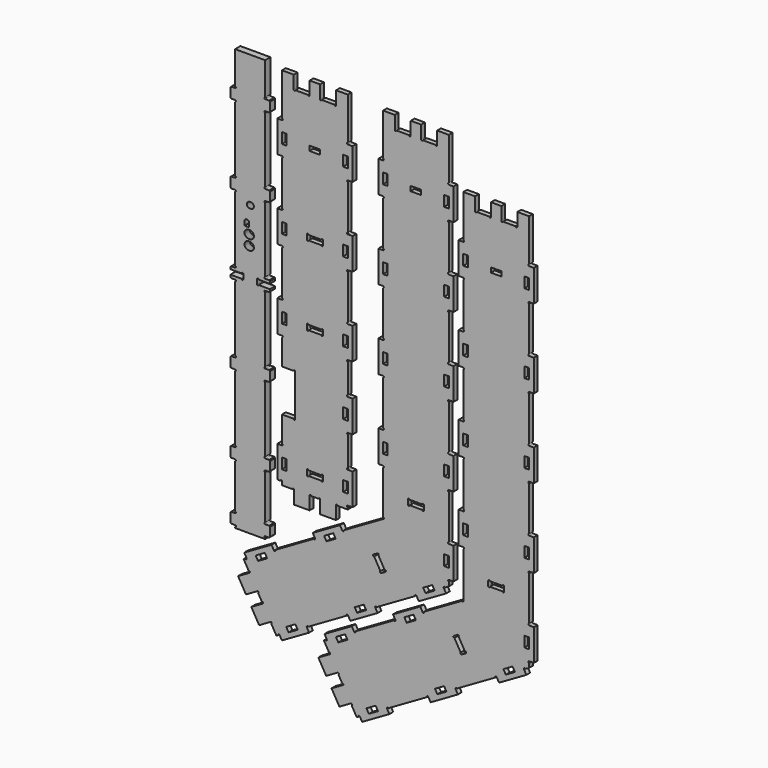
from build123d import *

# Parameters (mm, degrees)
F1_DEPTH = 25
F0_W     = 18
F0_H     = 40
F0_W_2   = 40
F0_H_2   = 18
F2_DEPTH = 18
F0_W_3   = 18.000018
F0_H_3   = 40.00004
F0_W_4   = 40.00004
F0_H_4   = 18.000018
F3_DEPTH = 18
F4_DEPTH = 18


# Not quite as in the source:
# - ends of sketch curves that miss each other by under 0.0002 mm in the source are joined


with BuildPart() as f1:
    # F0 (on Front) → F1 (new body)
    with BuildSketch(Plane.XZ):
        with BuildLine():
            Line((-423.791966, 1158.999877), (-537.792391, 1158.998909))
            Line((-537.792391, 1158.998909), (-537.791338, 1035.018779))
            ThreePointArc((-537.791338, 1035.0187789999), (-534.7813120001, 1032.0088045), (-537.791287, 1028.9987790001))
            Line((-537.791287, 1028.998779), (-552.791302, 1028.998346))
            Line((-552.791302, 1028.998346), (-555.79128, 1025.998623))
            Line((-555.79128, 1025.998623), (-555.790991, 991.998589))
            Line((-555.790991, 991.998589), (-552.790963, 988.998306))
            Line((-552.790963, 988.998306), (-537.790948, 988.998433))
            ThreePointArc((-537.790948, 988.9984329995), (-534.7808930005, 985.9884885), (-537.790837, 982.9784330005))
            Line((-537.790837, 982.978433), (-537.786301, 735.018479))
            ThreePointArc((-537.786301, 735.0184789995), (-534.7762460005, 732.008534), (-537.786191, 728.9984790005))
            Line((-537.786191, 728.998479), (-552.786206, 728.998046))
            Line((-552.786206, 728.998046), (-555.786184, 725.998323))
            Line((-555.786184, 725.998323), (-555.785895, 691.998289))
            Line((-555.785895, 691.998289), (-552.785866, 688.998006))
            Line((-552.785866, 688.998006), (-537.785851, 688.998133))
            ThreePointArc((-537.785851, 688.9981329997), (-534.7758110003, 685.988173), (-537.785771, 682.9781330003))
            Line((-537.785771, 682.978133), (-537.78245, 435.016937))
            ThreePointArc((-537.78245, 435.0169369997), (-534.7724100003, 432.0069775), (-537.782369, 428.9969370003))
            Line((-537.782369, 428.996937), (-552.782384, 428.996809))
            Line((-552.782384, 428.996809), (-555.782361, 425.997087))
            Line((-555.782361, 425.997087), (-555.783568, 417.996773))
            Line((-555.783568, 417.996773), (-512.803519, 417.997503))
            ThreePointArc((-512.8035189996, 417.997503), (-509.79357, 421.0075539996), (-506.7835190004, 417.997605))
            Line((-506.783519, 417.997605), (-506.783213, 399.997587))
            ThreePointArc((-506.7832130004, 399.997587), (-509.793162, 396.9875360004), (-512.8032129996, 399.997485))
            Line((-512.803213, 399.997485), (-555.783262, 399.996755))
            Line((-555.783262, 399.996755), (-555.782073, 391.996747))
            Line((-555.782073, 391.996747), (-552.782044, 388.996769))
            Line((-552.782044, 388.996769), (-537.782029, 388.996897))
            ThreePointArc((-537.782029, 388.9968969992), (-534.7719590008, 385.9869665), (-537.78189, 382.9768970008))
            Line((-537.78189, 382.976897), (-537.776138, 135.017879))
            ThreePointArc((-537.776138, 135.0178789992), (-534.7660680008, 132.0079485), (-537.775999, 128.9978790008))
            Line((-537.775999, 128.997879), (-552.776014, 128.997446))
            Line((-552.776014, 128.997446), (-555.775991, 125.997723))
            Line((-555.775991, 125.997723), (-555.775702, 91.997689))
            Line((-555.775702, 91.997689), (-552.775674, 88.997406))
            Line((-552.775674, 88.997406), (-537.775659, 88.997534))
            ThreePointArc((-537.775659, 88.9975339995), (-534.7656040005, 85.987589), (-537.775549, 82.9775340005))
            Line((-537.775549, 82.977534), (-537.771013, -164.982421))
            ThreePointArc((-537.771013, -164.9824210005), (-534.7609580005, -167.992366), (-537.770903, -171.0024209995))
            Line((-537.770903, -171.002421), (-552.770918, -171.002854))
            Line((-552.770918, -171.002854), (-555.770895, -174.002577))
            Line((-555.770895, -174.002577), (-555.770606, -208.002611))
            Line((-555.770606, -208.002611), (-552.770578, -211.002894))
            Line((-552.770578, -211.002894), (-537.770563, -211.002766))
            ThreePointArc((-537.770563, -211.0027660007), (-534.7604960008, -214.0126985), (-537.770428, -217.0227659992))
            Line((-537.770428, -217.022766), (-537.766657, -384.982641))
            ThreePointArc((-537.766657, -384.9826410007), (-534.7565900008, -387.9925735), (-537.766522, -391.0026409992))
            Line((-537.766522, -391.002641), (-552.766536, -391.003074))
            Line((-552.766536, -391.003074), (-555.766514, -394.002796))
            Line((-555.766514, -394.002796), (-555.766225, -428.00283))
            Line((-555.766225, -428.00283), (-552.766197, -431.003114))
            Line((-552.766197, -431.003114), (-537.766182, -431.002986))
            ThreePointArc((-537.766182, -431.002986001), (-534.756104001, -434.012908), (-537.766026, -437.022985999))
            Line((-537.766026, -437.022986), (-537.76593, -440.766858))
            Line((-537.76593, -440.766858), (-423.765503, -440.766858))
            Line((-423.765503, -440.766858), (-423.7656, -437.022018))
            ThreePointArc((-423.7656, -437.022017999), (-426.775677999, -434.012096), (-423.765756, -431.002018001))
            Line((-423.765756, -431.002018), (-408.765741, -431.001891))
            Line((-408.765741, -431.001891), (-405.765764, -428.001862))
            Line((-405.765764, -428.001862), (-405.766052, -394.001828))
            Line((-405.766052, -394.001828), (-408.766081, -391.001851))
            Line((-408.766081, -391.001851), (-423.766096, -391.001672))
            ThreePointArc((-423.766096, -391.0016719993), (-426.7761629992, -387.9917395), (-423.766231, -384.9816720008))
            Line((-423.766231, -384.981672), (-423.770002, -217.021798))
            ThreePointArc((-423.770002, -217.0217979993), (-426.7800689992, -214.0118655), (-423.770137, -211.0017980008))
            Line((-423.770137, -211.001798), (-408.770122, -211.001671))
            Line((-408.770122, -211.001671), (-405.770145, -208.001642))
            Line((-405.770145, -208.001642), (-405.770433, -174.001608))
            Line((-405.770433, -174.001608), (-408.770462, -171.001631))
            Line((-408.770462, -171.001631), (-423.770477, -171.001452))
            ThreePointArc((-423.770477, -171.0014519995), (-426.7805319995, -167.991507), (-423.770587, -164.9814520005))
            Line((-423.770587, -164.981452), (-423.775123, 82.978502))
            ThreePointArc((-423.775123, 82.9785020005), (-426.7851779995, 85.988447), (-423.775233, 88.9985019995))
            Line((-423.775233, 88.998502), (-408.775218, 88.998629))
            Line((-408.775218, 88.998629), (-405.775241, 91.998658))
            Line((-405.775241, 91.998658), (-405.77553, 125.998692))
            Line((-405.77553, 125.998692), (-408.775558, 128.998669))
            Line((-408.775558, 128.998669), (-423.775573, 128.998848))
            ThreePointArc((-423.775573, 128.9988480008), (-426.7856429992, 132.008778), (-423.775713, 135.0188479992))
            Line((-423.775713, 135.018848), (-423.781464, 382.977865))
            ThreePointArc((-423.781464, 382.9778650008), (-426.7915339992, 385.987795), (-423.781604, 388.9978649992))
            Line((-423.781604, 388.997865), (-408.781589, 388.997993))
            Line((-408.781589, 388.997993), (-405.781611, 391.998021))
            Line((-405.781611, 391.998021), (-405.784144, 399.999303))
            Line((-405.784144, 399.999303), (-448.764193, 399.998573))
            ThreePointArc((-448.7641930004, 399.998573), (-451.774142, 396.9885220004), (-454.7841929996, 399.998471))
            Line((-454.784193, 399.998471), (-454.784498, 417.998489))
            ThreePointArc((-454.7844979996, 417.998489), (-451.774549, 421.0085399996), (-448.7644980004, 417.998591))
            Line((-448.764498, 417.998591), (-405.784449, 417.999321))
            Line((-405.784449, 417.999321), (-405.7819, 425.998361))
            Line((-405.7819, 425.998361), (-408.781928, 428.998338))
            Line((-408.781928, 428.998338), (-423.781943, 428.997905))
            ThreePointArc((-423.781943, 428.9979050003), (-426.7919839997, 432.0078645), (-423.782024, 435.0179049997))
            Line((-423.782024, 435.017905), (-423.785345, 682.979102))
            ThreePointArc((-423.785345, 682.9791020003), (-426.7953849997, 685.9890615), (-423.785426, 688.9991019997))
            Line((-423.785426, 688.999102), (-408.785411, 688.999229))
            Line((-408.785411, 688.999229), (-405.785433, 691.999258))
            Line((-405.785433, 691.999258), (-405.785722, 725.999292))
            Line((-405.785722, 725.999292), (-408.78575, 728.999269))
            Line((-408.78575, 728.999269), (-423.785766, 728.999447))
            ThreePointArc((-423.785766, 728.9994470005), (-426.7958209995, 732.009392), (-423.785876, 735.0194469995))
            Line((-423.785876, 735.019447), (-423.790412, 982.979402))
            ThreePointArc((-423.790412, 982.9794020005), (-426.8004669995, 985.989347), (-423.790522, 988.9994019995))
            Line((-423.790522, 988.999402), (-408.790507, 988.999529))
            Line((-408.790507, 988.999529), (-405.790529, 991.999557))
            Line((-405.790529, 991.999557), (-405.790818, 1025.999591))
            Line((-405.790818, 1025.999591), (-408.790847, 1028.999569))
            Line((-408.790847, 1028.999569), (-423.790862, 1028.999747))
            ThreePointArc((-423.790862, 1028.9997470001), (-426.8008879999, 1032.0097215), (-423.790913, 1035.0197469999))
            Line((-423.790913, 1035.019747), (-423.791966, 1158.999877))
        make_face()
        Polygon((-466.588005, 519.290267), (-466.585583, 518.928201), (-466.582605, 518.560818), (-466.58894, 518.194219), (-466.604522, 517.828573), (-466.629283, 517.464048), (-466.663159, 517.100814), (-466.706082, 516.739038), (-466.757987, 516.378891), (-466.818807, 516.02054), (-466.888477, 515.664154), (-466.966929, 515.309903), (-467.054098, 514.957954), (-467.149917, 514.608477), (-467.254321, 514.26164), (-467.367243, 513.917612), (-467.488616, 513.576563), (-467.618375, 513.23866), (-467.756453, 512.904072), (-467.902785, 512.572969), (-468.057303, 512.245518), (-468.219942, 511.921889), (-468.390635, 511.602251), (-468.569317, 511.286772), (-468.755921, 510.975621), (-468.95038, 510.668967), (-469.152629, 510.366978), (-469.362601, 510.069824), (-469.580231, 509.777672), (-469.805451, 509.490693), (-470.038196, 509.209054), (-470.278399, 508.932924), (-470.525995, 508.662473), (-470.780917, 508.397868), (-471.113663, 508.09174), (-471.453327, 507.794659), (-471.799706, 507.506702), (-472.152593, 507.227947), (-472.511785, 506.958472), (-472.877077, 506.698355), (-473.248263, 506.447673), (-473.625141, 506.206503), (-474.007504, 505.974925), (-474.395148, 505.753015), (-474.787869, 505.540852), (-475.185462, 505.338513), (-475.587722, 505.146075), (-475.994444, 504.963617), (-476.405425, 504.791217), (-476.820458, 504.628951), (-477.239341, 504.476899), (-477.661867, 504.335137), (-478.087833, 504.203744), (-478.517033, 504.082796), (-478.949264, 503.972373), (-479.384319, 503.872551), (-479.821996, 503.783409), (-480.262089, 503.705024), (-480.704393, 503.637474), (-481.148703, 503.580837), (-481.594816, 503.53519), (-482.042527, 503.500611), (-482.49163, 503.477179), (-482.941921, 503.46497), (-483.393196, 503.464063), (-483.84525, 503.474535), (-484.336231, 503.460473), (-484.826397, 503.458917), (-485.315521, 503.469782), (-485.803377, 503.492983), (-486.289737, 503.528433), (-486.774376, 503.576048), (-487.257065, 503.635743), (-487.737578, 503.707431), (-488.215688, 503.791027), (-488.691169, 503.886445), (-489.163793, 503.993602), (-489.633334, 504.11241), (-490.099564, 504.242784), (-490.562258, 504.384639), (-491.021187, 504.53789), (-491.476125, 504.702451), (-491.926845, 504.878237), (-492.373121, 505.065162), (-492.814726, 505.26314), (-493.251432, 505.472087), (-493.683012, 505.691916), (-494.109241, 505.922543), (-494.529891, 506.163882), (-494.944734, 506.415847), (-495.353545, 506.678353), (-495.756097, 506.951315), (-496.152162, 507.234647), (-496.541514, 507.528264), (-496.923925, 507.83208), (-497.29917, 508.146009), (-497.66702, 508.469967), (-498.02725, 508.803868), (-498.28159, 509.053898), (-498.528749, 509.309936), (-498.768655, 509.571812), (-499.001239, 509.839353), (-499.226428, 510.112389), (-499.44415, 510.390747), (-499.654335, 510.674257), (-499.856911, 510.962748), (-500.051808, 511.256048), (-500.238952, 511.553986), (-500.418274, 511.85639), (-500.589701, 512.163089), (-500.753163, 512.473912), (-500.908588, 512.788687), (-501.055905, 513.107243), (-501.195042, 513.42941), (-501.325928, 513.755014), (-501.448491, 514.083886), (-501.562661, 514.415854), (-501.668367, 514.750746), (-501.765535, 515.088392), (-501.854096, 515.428619), (-501.933978, 515.771257), (-502.005109, 516.116134), (-502.067419, 516.463078), (-502.120836, 516.81192), (-502.165288, 517.162486), (-502.200704, 517.514607), (-502.227013, 517.86811), (-502.244143, 518.222824), (-502.252024, 518.578579), (-502.250583, 518.935201), (-502.247369, 519.297669), (-502.234713, 519.659142), (-502.212689, 520.019448), (-502.181372, 520.378414), (-502.140834, 520.735865), (-502.09115, 521.091629), (-502.032395, 521.445531), (-501.964641, 521.797399), (-501.887962, 522.147059), (-501.802433, 522.494338), (-501.708128, 522.839062), (-501.60512, 523.181057), (-501.493484, 523.52015), (-501.373293, 523.856168), (-501.244621, 524.188938), (-501.107542, 524.518285), (-500.96213, 524.844036), (-500.808459, 525.166018), (-500.646602, 525.484058), (-500.476635, 525.797981), (-500.29863, 526.107615), (-500.112662, 526.412786), (-499.918804, 526.713321), (-499.71713, 527.009045), (-499.507715, 527.299786), (-499.290632, 527.58537), (-499.065955, 527.865624), (-498.833758, 528.140375), (-498.594116, 528.409447), (-498.347101, 528.67267), (-498.092787, 528.929868), (-497.83125, 529.180868), (-497.472913, 529.504776), (-497.107237, 529.818882), (-496.734444, 530.123107), (-496.354756, 530.417371), (-495.968394, 530.701592), (-495.57558, 530.975691), (-495.176537, 531.239588), (-494.771484, 531.493201), (-494.360646, 531.736452), (-493.944242, 531.969258), (-493.522495, 532.191541), (-493.095627, 532.40322), (-492.663859, 532.604214), (-492.227413, 532.794443), (-491.786511, 532.973826), (-491.341375, 533.142285), (-490.892226, 533.299737), (-490.439286, 533.446103), (-489.982777, 533.581303), (-489.52292, 533.705256), (-489.059937, 533.817882), (-488.594051, 533.9191), (-488.125482, 534.008831), (-487.654453, 534.086993), (-487.181185, 534.153507), (-486.7059, 534.208292), (-486.22882, 534.251268), (-485.750166, 534.282355), (-485.27016, 534.301472), (-484.789025, 534.308539), (-484.306981, 534.303475), (-483.82425, 534.286201), (-483.373776, 534.293577), (-482.924179, 534.289508), (-482.475666, 534.274074), (-482.028445, 534.247355), (-481.582722, 534.209432), (-481.138706, 534.160386), (-480.696603, 534.100296), (-480.25662, 534.029243), (-479.818965, 533.947307), (-479.383844, 533.854569), (-478.951466, 533.751108), (-478.522037, 533.637006), (-478.095765, 533.512342), (-477.672856, 533.377197), (-477.253518, 533.231651), (-476.837958, 533.075785), (-476.426384, 532.909678), (-476.019002, 532.733411), (-475.61602, 532.547065), (-475.217645, 532.35072), (-474.824084, 532.144455), (-474.435545, 531.928352), (-474.052234, 531.702491), (-473.674359, 531.466951), (-473.302128, 531.221814), (-472.935746, 530.96716), (-472.575422, 530.703069), (-472.221363, 530.429621), (-471.873775, 530.146896), (-471.532867, 529.854976), (-471.198845, 529.55394), (-470.871917, 529.243868), (-470.617105, 528.9867), (-470.369403, 528.723681), (-470.12888, 528.454975), (-469.895603, 528.180748), (-469.669644, 527.901162), (-469.451069, 527.616383), (-469.239948, 527.326576), (-469.036349, 527.031904), (-468.840342, 526.732533), (-468.651994, 526.428627), (-468.471376, 526.12035), (-468.298555, 525.807866), (-468.133601, 525.491341), (-467.976582, 525.170938), (-467.827567, 524.846823), (-467.686625, 524.51916), (-467.553824, 524.188112), (-467.429234, 523.853846), (-467.312923, 523.516524), (-467.20496, 523.176313), (-467.105414, 522.833375), (-467.014353, 522.487876), (-466.931847, 522.13998), (-466.857964, 521.789852), (-466.792772, 521.437656), (-466.736341, 521.083557), (-466.68874, 520.727719), (-466.650037, 520.370306), (-466.620301, 520.011484), (-466.599601, 519.651416), align=None, mode=Mode.SUBTRACT)
        Polygon((-484.56625, 596.259535), (-484.56625, 580.896868), (-502.040583, 580.896868), (-502.040583, 596.259535), (-502.037605, 596.692113), (-502.012273, 597.12218), (-501.96493, 597.548917), (-501.895917, 597.971509), (-501.805575, 598.389137), (-501.694247, 598.800986), (-501.562275, 599.206238), (-501.41, 599.604076), (-501.237764, 599.993684), (-501.045909, 600.374245), (-500.834776, 600.744941), (-500.604708, 601.104957), (-500.356047, 601.453474), (-500.089133, 601.789676), (-499.804309, 602.112746), (-499.501917, 602.421868), (-499.194347, 602.719752), (-498.873284, 603.00069), (-498.539506, 603.26436), (-498.193792, 603.510441), (-497.836922, 603.738612), (-497.469674, 603.948552), (-497.09283, 604.139938), (-496.707167, 604.312451), (-496.313464, 604.465769), (-495.912503, 604.59957), (-495.50506, 604.713533), (-495.091917, 604.807337), (-494.673851, 604.88066), (-494.251643, 604.933182), (-493.826072, 604.96458), (-493.397917, 604.974535), (-492.959051, 604.977133), (-492.522379, 604.957149), (-492.088729, 604.914913), (-491.658927, 604.850759), (-491.233801, 604.765016), (-490.814178, 604.658017), (-490.400886, 604.530093), (-489.99475, 604.381576), (-489.596599, 604.212798), (-489.207259, 604.024089), (-488.827558, 603.815781), (-488.458323, 603.588207), (-488.100381, 603.341696), (-487.754559, 603.076582), (-487.421684, 602.793196), (-487.102583, 602.491868), (-486.801473, 602.176756), (-486.51786, 601.847959), (-486.252068, 601.506283), (-486.004422, 601.152535), (-485.775246, 600.787521), (-485.564867, 600.412048), (-485.373607, 600.026922), (-485.201792, 599.632951), (-485.049746, 599.230941), (-484.917795, 598.821699), (-484.806263, 598.40603), (-484.715474, 597.984743), (-484.645754, 597.558643), (-484.597426, 597.128537), (-484.570817, 596.695232), align=None, mode=Mode.SUBTRACT)
        Polygon((-466.588005, 558.004933), (-466.585583, 557.642868), (-466.582605, 557.275485), (-466.58894, 556.908886), (-466.604522, 556.54324), (-466.629283, 556.178715), (-466.663159, 555.815481), (-466.706082, 555.453705), (-466.757987, 555.093558), (-466.818807, 554.735207), (-466.888477, 554.378821), (-466.966929, 554.024569), (-467.054098, 553.672621), (-467.149917, 553.323143), (-467.254321, 552.976307), (-467.367243, 552.632279), (-467.488616, 552.291229), (-467.618375, 551.953326), (-467.756453, 551.618739), (-467.902785, 551.287635), (-468.057303, 550.960185), (-468.219942, 550.636556), (-468.390635, 550.316918), (-468.569317, 550.001439), (-468.755921, 549.690288), (-468.95038, 549.383634), (-469.152629, 549.081645), (-469.362601, 548.78449), (-469.580231, 548.492339), (-469.805451, 548.20536), (-470.038196, 547.923721), (-470.278399, 547.647591), (-470.525995, 547.377139), (-470.780917, 547.112535), (-471.113663, 546.806407), (-471.453327, 546.509326), (-471.799706, 546.221369), (-472.152593, 545.942614), (-472.511785, 545.673139), (-472.877077, 545.413021), (-473.248263, 545.162339), (-473.625141, 544.92117), (-474.007504, 544.689592), (-474.395148, 544.467682), (-474.787869, 544.255519), (-475.185462, 544.053179), (-475.587722, 543.860742), (-475.994444, 543.678284), (-476.405425, 543.505883), (-476.820458, 543.343618), (-477.239341, 543.191566), (-477.661867, 543.049804), (-478.087833, 542.91841), (-478.517033, 542.797463), (-478.949264, 542.68704), (-479.384319, 542.587218), (-479.821996, 542.498076), (-480.262089, 542.419691), (-480.704393, 542.352141), (-481.148703, 542.295504), (-481.594816, 542.249857), (-482.042527, 542.215278), (-482.49163, 542.191846), (-482.941921, 542.179637), (-483.393196, 542.178729), (-483.84525, 542.189201), (-484.336231, 542.175139), (-484.826397, 542.173584), (-485.315521, 542.184449), (-485.803377, 542.207649), (-486.289737, 542.2431), (-486.774376, 542.290715), (-487.257065, 542.350409), (-487.737578, 542.422097), (-488.215688, 542.505693), (-488.691169, 542.601112), (-489.163793, 542.708268), (-489.633334, 542.827076), (-490.099564, 542.957451), (-490.562258, 543.099306), (-491.021187, 543.252557), (-491.476125, 543.417118), (-491.926845, 543.592904), (-492.373121, 543.779828), (-492.814726, 543.977807), (-493.251432, 544.186753), (-493.683012, 544.406583), (-494.109241, 544.63721), (-494.529891, 544.878549), (-494.944734, 545.130514), (-495.353545, 545.39302), (-495.756097, 545.665982), (-496.152162, 545.949314), (-496.541514, 546.242931), (-496.923925, 546.546746), (-497.29917, 546.860676), (-497.66702, 547.184634), (-498.02725, 547.518535), (-498.28159, 547.768565), (-498.528749, 548.024603), (-498.768655, 548.286479), (-499.001239, 548.55402), (-499.226428, 548.827055), (-499.44415, 549.105414), (-499.654335, 549.388924), (-499.856911, 549.677415), (-500.051808, 549.970715), (-500.238952, 550.268652), (-500.418274, 550.571056), (-500.589701, 550.877755), (-500.753163, 551.188578), (-500.908588, 551.503354), (-501.055905, 551.82191), (-501.195042, 552.144076), (-501.325928, 552.469681), (-501.448491, 552.798553), (-501.562661, 553.130521), (-501.668367, 553.465413), (-501.765535, 553.803058), (-501.854096, 554.143286), (-501.933978, 554.485923), (-502.005109, 554.8308), (-502.067419, 555.177745), (-502.120836, 555.526587), (-502.165288, 555.877153), (-502.200704, 556.229274), (-502.227013, 556.582777), (-502.244143, 556.937491), (-502.252024, 557.293245), (-502.250583, 557.649868), (-502.247369, 558.012335), (-502.234713, 558.373809), (-502.212689, 558.734115), (-502.181372, 559.09308), (-502.140834, 559.450532), (-502.09115, 559.806295), (-502.032395, 560.160198), (-501.964641, 560.512066), (-501.887962, 560.861726), (-501.802433, 561.209005), (-501.708128, 561.553728), (-501.60512, 561.895723), (-501.493484, 562.234817), (-501.373293, 562.570835), (-501.244621, 562.903604), (-501.107542, 563.232951), (-500.96213, 563.558703), (-500.808459, 563.880685), (-500.646602, 564.198724), (-500.476635, 564.512648), (-500.29863, 564.822282), (-500.112662, 565.127453), (-499.918804, 565.427987), (-499.71713, 565.723712), (-499.507715, 566.014453), (-499.290632, 566.300037), (-499.065955, 566.580291), (-498.833758, 566.855041), (-498.594116, 567.124114), (-498.347101, 567.387336), (-498.092787, 567.644534), (-497.83125, 567.895535), (-497.472913, 568.219442), (-497.107237, 568.533549), (-496.734444, 568.837774), (-496.354756, 569.132037), (-495.968394, 569.416259), (-495.57558, 569.690358), (-495.176537, 569.954254), (-494.771484, 570.207868), (-494.360646, 570.451118), (-493.944242, 570.683925), (-493.522495, 570.906208), (-493.095627, 571.117886), (-492.663859, 571.31888), (-492.227413, 571.509109), (-491.786511, 571.688493), (-491.341375, 571.856951), (-490.892226, 572.014404), (-490.439286, 572.16077), (-489.982777, 572.29597), (-489.52292, 572.419923), (-489.059937, 572.532548), (-488.594051, 572.633767), (-488.125482, 572.723497), (-487.654453, 572.80166), (-487.181185, 572.868174), (-486.7059, 572.922959), (-486.22882, 572.965935), (-485.750166, 572.997022), (-485.27016, 573.016139), (-484.789025, 573.023206), (-484.306981, 573.018142), (-483.82425, 573.000868), (-483.373776, 573.008244), (-482.924179, 573.004174), (-482.475666, 572.98874), (-482.028445, 572.962022), (-481.582722, 572.924099), (-481.138706, 572.875053), (-480.696603, 572.814963), (-480.25662, 572.74391), (-479.818965, 572.661974), (-479.383844, 572.569236), (-478.951466, 572.465775), (-478.522037, 572.351673), (-478.095765, 572.227009), (-477.672856, 572.091864), (-477.253518, 571.946318), (-476.837958, 571.790451), (-476.426384, 571.624345), (-476.019002, 571.448078), (-475.61602, 571.261732), (-475.217645, 571.065386), (-474.824084, 570.859122), (-474.435545, 570.643019), (-474.052234, 570.417157), (-473.674359, 570.181618), (-473.302128, 569.936481), (-472.935746, 569.681827), (-472.575422, 569.417735), (-472.221363, 569.144287), (-471.873775, 568.861563), (-471.532867, 568.569642), (-471.198845, 568.268606), (-470.871917, 567.958535), (-470.617105, 567.701367), (-470.369403, 567.438348), (-470.12888, 567.169642), (-469.895603, 566.895414), (-469.669644, 566.615829), (-469.451069, 566.33105), (-469.239948, 566.041243), (-469.036349, 565.746571), (-468.840342, 565.4472), (-468.651994, 565.143293), (-468.471376, 564.835016), (-468.298555, 564.522533), (-468.133601, 564.206008), (-467.976582, 563.885605), (-467.827567, 563.56149), (-467.686625, 563.233826), (-467.553824, 562.902779), (-467.429234, 562.568512), (-467.312923, 562.231191), (-467.20496, 561.890979), (-467.105414, 561.548042), (-467.014353, 561.202543), (-466.931847, 560.854647), (-466.857964, 560.504519), (-466.792772, 560.152323), (-466.736341, 559.798224), (-466.68874, 559.442385), (-466.650037, 559.084973), (-466.620301, 558.72615), (-466.599601, 558.366082), align=None, mode=Mode.SUBTRACT)
        Polygon((-466.658849, 656.582723), (-466.641583, 656.067535), (-466.640561, 655.552322), (-466.666106, 655.039834), (-466.717826, 654.531043), (-466.795328, 654.026925), (-466.898219, 653.528454), (-467.026105, 653.036603), (-467.178593, 652.552347), (-467.355292, 652.07666), (-467.555806, 651.610515), (-467.779744, 651.154888), (-468.026712, 650.710752), (-468.296318, 650.279082), (-468.588167, 649.86085), (-468.901868, 649.457033), (-469.237026, 649.068603), (-469.59325, 648.696535), (-469.849479, 648.438401), (-470.111859, 648.187737), (-470.380211, 647.944614), (-470.654356, 647.709106), (-470.934115, 647.481285), (-471.219309, 647.261224), (-471.509759, 647.048994), (-471.805286, 646.84467), (-472.105711, 646.648323), (-472.410855, 646.460027), (-472.720539, 646.279853), (-473.034584, 646.107875), (-473.352811, 645.944164), (-473.67504, 645.788795), (-474.001093, 645.641838), (-474.330792, 645.503368), (-474.663956, 645.373456), (-475.000406, 645.252176), (-475.339965, 645.139599), (-475.682452, 645.035799), (-476.02769, 644.940848), (-476.375497, 644.854819), (-476.725697, 644.777784), (-477.078109, 644.709816), (-477.432555, 644.650988), (-477.788856, 644.601372), (-478.146832, 644.561041), (-478.506305, 644.530067), (-478.867096, 644.508524), (-479.229025, 644.496483), (-479.591914, 644.494018), (-479.955583, 644.501201), (-480.317649, 644.487151), (-480.679239, 644.482147), (-481.04019, 644.486131), (-481.40034, 644.499046), (-481.759529, 644.520832), (-482.117594, 644.55143), (-482.474372, 644.590783), (-482.829703, 644.638832), (-483.183424, 644.695517), (-483.535373, 644.760782), (-483.885388, 644.834566), (-484.233308, 644.916813), (-484.57897, 645.007462), (-484.922213, 645.106456), (-485.262874, 645.213736), (-485.600792, 645.329243), (-485.935804, 645.452919), (-486.26775, 645.584706), (-486.596466, 645.724545), (-486.921791, 645.872376), (-487.243563, 646.028143), (-487.561621, 646.191786), (-487.875801, 646.363247), (-488.185943, 646.542467), (-488.491884, 646.729388), (-488.793462, 646.92395), (-489.090516, 647.126097), (-489.382883, 647.335768), (-489.670402, 647.552906), (-489.952911, 647.777453), (-490.230248, 648.009348), (-490.50225, 648.248535), (-490.866408, 648.651294), (-491.209642, 649.069722), (-491.531588, 649.502916), (-491.831885, 649.949972), (-492.110171, 650.40999), (-492.366082, 650.882066), (-492.599257, 651.365298), (-492.809333, 651.858785), (-492.995949, 652.361623), (-493.158741, 652.87291), (-493.297347, 653.391744), (-493.411406, 653.917222), (-493.500555, 654.448443), (-493.564431, 654.984503), (-493.602672, 655.524501), (-493.614917, 656.067535), (-493.589513, 656.593374), (-493.536376, 657.114951), (-493.455991, 657.63123), (-493.348844, 658.141175), (-493.215419, 658.643752), (-493.056202, 659.137923), (-492.871678, 659.622655), (-492.662333, 660.09691), (-492.428652, 660.559653), (-492.171121, 661.009849), (-491.890224, 661.446462), (-491.586448, 661.868457), (-491.260277, 662.274797), (-490.912197, 662.664447), (-490.542693, 663.036371), (-490.15225, 663.389535), (-489.894092, 663.629773), (-489.630298, 663.862633), (-489.361039, 664.088052), (-489.086491, 664.305965), (-488.806826, 664.516309), (-488.522217, 664.71902), (-488.232839, 664.914035), (-487.938865, 665.10129), (-487.640467, 665.280721), (-487.33782, 665.452265), (-487.031098, 665.615857), (-486.720473, 665.771435), (-486.406118, 665.918935), (-486.088209, 666.058292), (-485.766917, 666.189444), (-485.442417, 666.312326), (-485.114881, 666.426876), (-484.784484, 666.533029), (-484.451398, 666.630721), (-484.115798, 666.719889), (-483.777857, 666.80047), (-483.437747, 666.8724), (-483.095643, 666.935614), (-482.751719, 666.99005), (-482.406147, 667.035644), (-482.0591, 667.072332), (-481.710754, 667.10005), (-481.36128, 667.118735), (-481.010853, 667.128322), (-480.659645, 667.12875), (-480.307831, 667.119953), (-479.955583, 667.101868), (-479.605809, 667.113567), (-479.256593, 667.116331), (-478.908098, 667.110217), (-478.560487, 667.095287), (-478.213922, 667.0716), (-477.868565, 667.039217), (-477.524578, 666.998196), (-477.182125, 666.948597), (-476.841367, 666.890481), (-476.502466, 666.823907), (-476.165586, 666.748936), (-475.830888, 666.665626), (-475.498535, 666.574038), (-475.168688, 666.474231), (-474.841512, 666.366266), (-474.517167, 666.250201), (-474.195816, 666.126098), (-473.877621, 665.994015), (-473.562746, 665.854013), (-473.251352, 665.706152), (-472.943601, 665.55049), (-472.639656, 665.387089), (-472.339679, 665.216007), (-472.043833, 665.037306), (-471.75228, 664.851043), (-471.465183, 664.65728), (-471.182703, 664.456076), (-470.905003, 664.24749), (-470.632245, 664.031584), (-470.364592, 663.808416), (-470.102206, 663.578046), (-469.84525, 663.340535), (-469.476891, 662.979975), (-469.128971, 662.602431), (-468.801915, 662.208857), (-468.496146, 661.800207), (-468.212088, 661.377433), (-467.950164, 660.94149), (-467.710799, 660.493331), (-467.494417, 660.03391), (-467.30144, 659.56418), (-467.132294, 659.085095), (-466.987402, 658.597609), (-466.867187, 658.102675), (-466.772075, 657.601247), (-466.702487, 657.094279), align=None, mode=Mode.SUBTRACT)
    extrude(amount=F1_DEPTH)


with BuildPart() as f2:
    # F0 (on Front) → F2 (new body)
    with BuildSketch(Plane.XZ):
        with BuildLine():
            Line((-98.056252, -231.408427), (-98.056252, -111.908427))
            Line((-98.056252, -111.908427), (-116.05625, -111.908427))
            ThreePointArc((-116.05625, -111.908427), (-119.0662759999, -108.898453), (-116.056302, -105.8884270001))
            Line((-116.056302, -105.8884270001), (-116.057276, 5.88976))
            ThreePointArc((-116.057276, 5.88976), (-119.0673019999, 8.8997335), (-116.057329, 11.9097599999))
            Line((-116.057329, 11.9097599999), (-98.057442, 11.90976))
            Line((-98.057442, 11.90976), (-98.057442, 131.409838))
            Line((-98.057442, 131.409838), (-116.057325, 131.409838))
            ThreePointArc((-116.057325, 131.409838), (-119.067344, 134.419819), (-116.057363, 137.429838))
            Line((-116.057363, 137.429838), (-116.058073, 249.209176))
            ThreePointArc((-116.058073, 249.209176), (-119.068092, 252.219157), (-116.058111, 255.229176))
            Line((-116.058111, 255.229176), (-98.058109, 255.229176))
            Line((-98.058109, 255.229176), (-98.058109, 374.729176))
            Line((-98.058109, 374.729176), (-116.058109, 374.729176))
            ThreePointArc((-116.058109, 374.729176), (-119.068109, 377.739176), (-116.058109, 380.749176))
            Line((-116.058109, 380.749176), (-116.058109, 549.209176))
            ThreePointArc((-116.058109, 549.209176), (-119.068109, 552.219176), (-116.058109, 555.229176))
            Line((-116.058109, 555.229176), (-98.058109, 555.229176))
            Line((-98.058109, 555.229176), (-98.058109, 674.729176))
            Line((-98.058109, 674.729176), (-116.058109, 674.729176))
            ThreePointArc((-116.058109, 674.729176), (-119.068109, 677.739176), (-116.058109, 680.749176))
            Line((-116.058109, 680.749176), (-116.058109, 849.209176))
            ThreePointArc((-116.058109, 849.209176), (-119.068109, 852.219176), (-116.058109, 855.229176))
            Line((-116.058109, 855.229176), (-98.058109, 855.229176))
            Line((-98.058109, 855.229176), (-98.058109, 974.729176))
            Line((-98.058109, 974.729176), (-116.058111, 974.729176))
            ThreePointArc((-116.058111, 974.729176), (-119.068087, 977.7392), (-116.058063, 980.749176))
            Line((-116.058063, 980.749176), (-116.056776, 1141.424258))
            Line((-116.056776, 1141.424258), (-160.556774, 1141.424258))
            Line((-160.556774, 1141.424258), (-160.556774, 1091.424258))
            ThreePointArc((-160.556774, 1091.424258), (-163.566774, 1088.414258), (-166.576774, 1091.424258))
            Line((-166.576774, 1091.424258), (-215.036774, 1091.424258))
            ThreePointArc((-215.036774, 1091.424258), (-218.046774, 1088.414258), (-221.056774, 1091.424258))
            Line((-221.056774, 1091.424258), (-221.056774, 1141.424258))
            Line((-221.056774, 1141.424258), (-260.556774, 1141.424258))
            Line((-260.556774, 1141.424258), (-260.556774, 1091.424258))
            ThreePointArc((-260.556774, 1091.424258), (-263.566774, 1088.414258), (-266.576774, 1091.424258))
            Line((-266.576774, 1091.424258), (-315.036774, 1091.424258))
            ThreePointArc((-315.036774, 1091.424258), (-318.046774, 1088.414258), (-321.056774, 1091.424258))
            Line((-321.056774, 1091.424258), (-321.056774, 1141.424258))
            Line((-321.056774, 1141.424258), (-365.556776, 1141.424258))
            Line((-365.556776, 1141.424258), (-365.558063, 980.749176))
            ThreePointArc((-365.558063, 980.749176), (-362.548087, 977.739152), (-365.558111, 974.729176))
            Line((-365.558111, 974.729176), (-383.558109, 974.729176))
            Line((-383.558109, 974.729176), (-383.558109, 855.229176))
            Line((-383.558109, 855.229176), (-365.558109, 855.229176))
            ThreePointArc((-365.558109, 855.229176), (-362.548109, 852.219176), (-365.558109, 849.209176))
            Line((-365.558109, 849.209176), (-365.558109, 680.749176))
            ThreePointArc((-365.558109, 680.749176), (-362.548109, 677.739176), (-365.558109, 674.729176))
            Line((-365.558109, 674.729176), (-383.558109, 674.729176))
            Line((-383.558109, 674.729176), (-383.558109, 555.229176))
            Line((-383.558109, 555.229176), (-365.558109, 555.229176))
            ThreePointArc((-365.558109, 555.229176), (-362.548109, 552.219176), (-365.558109, 549.209176))
            Line((-365.558109, 549.209176), (-365.558109, 380.749176))
            ThreePointArc((-365.558109, 380.749176), (-362.548109, 377.739176), (-365.558109, 374.729176))
            Line((-365.558109, 374.729176), (-383.558109, 374.729176))
            Line((-383.558109, 374.729176), (-383.558109, 255.229176))
            Line((-383.558109, 255.229176), (-365.558111, 255.229176))
            ThreePointArc((-365.558111, 255.229176), (-362.548091, 252.2191965), (-365.55807, 249.209176))
            Line((-365.55807, 249.209176), (-365.557362, 151.911505))
            Line((-365.557362, 151.911505), (-321.575894, 151.911505))
            ThreePointArc((-321.575894, 151.911505), (-318.566628, 154.920771), (-315.557362, 151.911505))
            Line((-315.557362, 151.911505), (-315.557362, -8.088495))
            ThreePointArc((-315.557362, -8.088495), (-318.3682489999, -10.9001859713), (-321.1799399713, -8.0892990001))
            Line((-321.1799399713, -8.0892990001), (-365.557312, -8.088495))
            Line((-365.557312, -8.088495), (-365.556311, -105.888427))
            ThreePointArc((-365.556311, -105.888427), (-362.5462800002, -108.898396), (-365.556249, -111.9084269998))
            Line((-365.556249, -111.9084269998), (-383.556252, -111.908427))
            Line((-383.556252, -111.908427), (-383.556252, -231.408427))
            Line((-383.556252, -231.408427), (-371.576242, -231.408427))
            ThreePointArc((-371.576242, -231.408427), (-368.566242, -228.398427), (-365.556242, -231.408427))
            Line((-365.556242, -231.408427), (-365.556765, -244.71304))
            Line((-365.556765, -244.71304), (-326.576774, -244.71304))
            ThreePointArc((-326.576774, -244.71304), (-323.566774, -241.70304), (-320.556774, -244.71304))
            Line((-320.556774, -244.71304), (-320.556774, -294.71304))
            Line((-320.556774, -294.71304), (-261.056774, -294.71304))
            Line((-261.056774, -294.71304), (-261.056774, -244.71304))
            ThreePointArc((-261.056774, -244.71304), (-258.046774, -241.70304), (-255.036774, -244.71304))
            Line((-255.036774, -244.71304), (-226.576774, -244.71304))
            ThreePointArc((-226.576774, -244.71304), (-223.566774, -241.70304), (-220.556774, -244.71304))
            Line((-220.556774, -244.71304), (-220.556774, -294.71304))
            Line((-220.556774, -294.71304), (-161.056774, -294.71304))
            Line((-161.056774, -294.71304), (-161.056774, -244.71304))
            ThreePointArc((-161.056774, -244.71304), (-158.046774, -241.70304), (-155.036774, -244.71304))
            Line((-155.036774, -244.71304), (-116.056765, -244.71304))
            Line((-116.056765, -244.71304), (-116.056479, -237.428427))
            ThreePointArc((-116.056479, -237.428427), (-119.0663609977, -234.4183085), (-116.056242, -231.4084270024))
            Line((-116.056242, -231.4084270024), (-98.056252, -231.408427))
        make_face()
        with Locations((-356.806252, -171.658427)):
            Rectangle(F0_W, F0_H, mode=Mode.SUBTRACT)
        with BuildLine():
            Line((-265.038109, -162.408427), (-216.578109, -162.408427))
            ThreePointArc((-216.578109, -162.408427), (-213.568109, -159.398427), (-210.558109, -162.408427))
            Line((-210.558109, -162.408427), (-210.558109, -180.908427))
            ThreePointArc((-210.558109, -180.908427), (-213.568109, -183.918427), (-216.578109, -180.908427))
            Line((-216.578109, -180.908427), (-265.038109, -180.908427))
            ThreePointArc((-265.038109, -180.908427), (-268.048109, -183.918427), (-271.058109, -180.908427))
            Line((-271.058109, -180.908427), (-271.058109, -162.408427))
            ThreePointArc((-271.058109, -162.408427), (-268.048109, -159.398427), (-265.038109, -162.408427))
        make_face(mode=Mode.SUBTRACT)
        with Locations((-124.806252, -171.658427)):
            Rectangle(F0_W, F0_H, mode=Mode.SUBTRACT)
        with Locations((-356.808109, 314.979176)):
            Rectangle(F0_W, F0_H, mode=Mode.SUBTRACT)
        with Locations((-124.808109, 71.659799)):
            Rectangle(F0_W, F0_H, mode=Mode.SUBTRACT)
        with BuildLine():
            Line((-265.038109, 324.229176), (-216.578109, 324.229176))
            ThreePointArc((-216.578109, 324.229176), (-213.568109, 327.239176), (-210.558109, 324.229176))
            Line((-210.558109, 324.229176), (-210.558109, 305.729176))
            ThreePointArc((-210.558109, 305.729176), (-213.568109, 302.719176), (-216.578109, 305.729176))
            Line((-216.578109, 305.729176), (-265.038109, 305.729176))
            ThreePointArc((-265.038109, 305.729176), (-268.048109, 302.719176), (-271.058109, 305.729176))
            Line((-271.058109, 305.729176), (-271.058109, 324.229176))
            ThreePointArc((-271.058109, 324.229176), (-268.048109, 327.239176), (-265.038109, 324.229176))
        make_face(mode=Mode.SUBTRACT)
        with Locations((-124.808109, 314.979176)):
            Rectangle(F0_W, F0_H, mode=Mode.SUBTRACT)
        with Locations((-356.808109, 614.979176)):
            Rectangle(F0_W, F0_H, mode=Mode.SUBTRACT)
        with Locations((-356.808109, 914.979176)):
            Rectangle(F0_W, F0_H, mode=Mode.SUBTRACT)
        with BuildLine():
            Line((-265.038109, 624.229176), (-216.578109, 624.229176))
            ThreePointArc((-216.578109, 624.229176), (-213.568109, 627.239176), (-210.558109, 624.229176))
            Line((-210.558109, 624.229176), (-210.558109, 605.729176))
            ThreePointArc((-210.558109, 605.729176), (-213.568109, 602.719176), (-216.578109, 605.729176))
            Line((-216.578109, 605.729176), (-265.038109, 605.729176))
            ThreePointArc((-265.038109, 605.729176), (-268.048109, 602.719176), (-271.058109, 605.729176))
            Line((-271.058109, 605.729176), (-271.058109, 624.229176))
            ThreePointArc((-271.058109, 624.229176), (-268.048109, 627.239176), (-265.038109, 624.229176))
        make_face(mode=Mode.SUBTRACT)
        with Locations((-124.808109, 614.979176)):
            Rectangle(F0_W, F0_H, mode=Mode.SUBTRACT)
        with Locations((-240.808109, 914.979176)):
            Rectangle(F0_W_2, F0_H_2, mode=Mode.SUBTRACT)
        with Locations((-124.808109, 914.979176)):
            Rectangle(F0_W, F0_H, mode=Mode.SUBTRACT)
    extrude(amount=F2_DEPTH)


with BuildPart() as f3:
    # F0 (on Front) → F3 (new body)
    with BuildSketch(Plane.XZ):
        with BuildLine():
            Line((17.840502, 238.935062), (17.840609, 71.474882))
            ThreePointArc((17.840609, 71.474882), (20.8578738635, 68.0943984195), (17.5906129999, 64.9548819137))
            Line((17.5906129999, 64.9548819137), (-0.159463, 64.95489))
            Line((-0.159463, 64.95489), (-0.15952, -54.545221))
            Line((-0.15952, -54.545221), (17.590556, -54.545229))
            ThreePointArc((17.590556, -54.545229), (20.8482544886, -57.6851093406), (17.8405569631, -61.0652285294))
            Line((17.8405569631, -61.0652285294), (17.840596, -226.417026))
            ThreePointArc((17.840596, -226.417026), (20.8589435838, -229.7643172278), (17.6575850038, -232.9370261999))
            Line((17.6575850038, -232.9370261999), (-130.916136, -318.716168))
            ThreePointArc((-130.916136, -318.716168), (-132.3350894791, -323.0194378193), (-136.6876207696, -321.7596638675))
            Line((-136.6876207696, -321.7596638675), (-145.562651, -306.387643))
            Line((-145.562651, -306.387643), (-249.052864, -366.137679))
            Line((-249.052864, -366.137679), (-240.177834, -381.509699))
            ThreePointArc((-240.177834, -381.509699), (-241.268201543, -385.9008891217), (-245.6993194407, -384.9862056159))
            Line((-245.6993194407, -384.9862056159), (-390.724063, -468.716281))
            ThreePointArc((-390.724063, -468.716281), (-392.1430184528, -473.0195503328), (-396.4955492019, -471.7597751161))
            Line((-396.4955492019, -471.7597751161), (-405.370558, -456.387808))
            Line((-405.370558, -456.387808), (-508.860698, -516.137868))
            Line((-508.860698, -516.137868), (-499.985682, -531.509846))
            ThreePointArc((-499.985682, -531.509846), (-501.0765041427, -535.9009229239), (-505.5075270402, -534.9857820276))
            Line((-505.5075270402, -534.9857820276), (-511.384503, -538.37803))
            Line((-511.384503, -538.37803), (-492.14377, -571.703932))
            ThreePointArc((-492.14377, -571.703932), (-487.8405009705, -573.1228858776), (-489.1002751325, -577.4754167696))
            Line((-489.1002751325, -577.4754167696), (-532.185082, -602.350442))
            Line((-532.185082, -602.350442), (-502.435052, -653.879005))
            Line((-502.435052, -653.879005), (-459.350245, -629.00398))
            ThreePointArc((-459.350245, -629.00398), (-454.9590548783, -630.094347543), (-455.8737383841, -634.5254654407))
            Line((-455.8737383841, -634.5254654407), (-442.144431, -658.305323))
            ThreePointArc((-442.144431, -658.305323), (-437.8411624571, -659.7242788513), (-439.1009378839, -664.0768092019))
            Line((-439.1009378839, -664.0768092019), (-482.185757, -688.951841))
            Line((-482.185757, -688.951841), (-452.435014, -740.48164))
            Line((-452.435014, -740.48164), (-409.350195, -715.606607))
            ThreePointArc((-409.350195, -715.606607), (-404.959005295, -716.6969764695), (-405.8736900636, -721.1280939073))
            Line((-405.8736900636, -721.1280939073), (-386.63369, -754.452776))
            Line((-386.63369, -754.452776), (-380.757049, -751.059896))
            ThreePointArc((-380.757049, -751.059896), (-379.338094739, -746.7566267684), (-374.9855637981, -748.0164018839))
            Line((-374.9855637981, -748.0164018839), (-366.110555, -763.388369))
            Line((-366.110555, -763.388369), (-262.620415, -703.638309))
            Line((-262.620415, -703.638309), (-271.495424, -688.266342))
            ThreePointArc((-271.495424, -688.266342), (-270.4050570453, -683.8751522488), (-265.9739393464, -684.7898342379))
            Line((-265.9739393464, -684.7898342379), (-120.949163, -601.059678))
            ThreePointArc((-120.949163, -601.059678), (-119.5302091224, -596.7564089705), (-115.1776782304, -598.0161831325))
            Line((-115.1776782304, -598.0161831325), (-106.302648, -613.388204))
            Line((-106.302648, -613.388204), (-2.812487, -553.638198))
            Line((-2.812487, -553.638198), (-11.687517, -538.266177))
            ThreePointArc((-11.687517, -538.266177), (-10.5971490903, -533.8749876474), (-6.1660315593, -534.7896713841))
            Line((-6.1660315593, -534.7896713841), (138.858609, -451.059656))
            ThreePointArc((138.858609, -451.059656), (140.277563261, -446.7563867684), (144.6300942019, -448.0161618839))
            Line((144.6300942019, -448.0161618839), (153.505103, -463.388129))
            Line((153.505103, -463.388129), (256.995243, -403.638069))
            Line((256.995243, -403.638069), (248.120234, -388.266102))
            ThreePointArc((248.120234, -388.266102), (249.2106019097, -383.8749126474), (253.6417194407, -384.7895963841))
            Line((253.6417194407, -384.7895963841), (267.340917, -376.880359))
            Line((267.340917, -376.880359), (267.34091, -361.06529))
            ThreePointArc((267.34091, -361.06529), (264.3236451542, -357.6848049574), (267.5909070001, -354.5452889152))
            Line((267.5909070001, -354.5452889152), (285.340925, -354.545281))
            Line((285.340925, -354.545281), (285.340867, -235.04516))
            Line((285.340867, -235.04516), (267.590849, -235.045109))
            ThreePointArc((267.590849, -235.045109), (264.3331495497, -231.9052296571), (267.3408460429, -228.5251095484))
            Line((267.3408460429, -228.5251095484), (267.340752, -61.065221))
            ThreePointArc((267.340752, -61.065221), (264.3234871365, -57.6847374195), (267.5907480001, -54.5452209137))
            Line((267.5907480001, -54.5452209137), (285.340824, -54.545229))
            Line((285.340824, -54.545229), (285.340881, 64.954942))
            Line((285.340881, 64.954942), (267.590806, 64.954951))
            ThreePointArc((267.590806, 64.954951), (264.333107532, 68.0948308035), (267.3408039651, 71.4749504455))
            Line((267.3408039651, 71.4749504455), (267.34075, 238.935079))
            ThreePointArc((267.34075, 238.935079), (264.3234861748, 242.3155635783), (267.5907480001, 245.4550790848))
            Line((267.5907480001, 245.4550790848), (285.340824, 245.455071))
            Line((285.340824, 245.455071), (285.340881, 364.955242))
            Line((285.340881, 364.955242), (267.590806, 364.955251))
            ThreePointArc((267.590806, 364.955251), (264.333107532, 368.0951308035), (267.3408039651, 371.4752504455))
            Line((267.3408039651, 371.4752504455), (267.34075, 538.935379))
            ThreePointArc((267.34075, 538.935379), (264.3234861748, 542.3158635783), (267.5907480001, 545.4553790848))
            Line((267.5907480001, 545.4553790848), (285.340824, 545.455371))
            Line((285.340824, 545.455371), (285.340881, 664.955542))
            Line((285.340881, 664.955542), (267.590806, 664.955551))
            ThreePointArc((267.590806, 664.955551), (264.3331084923, 668.0954318403), (267.3408060369, 671.4755505294))
            Line((267.3408060369, 671.4755505294), (267.340806, 838.935701))
            ThreePointArc((267.340806, 838.935701), (264.3235432131, 842.3161865762), (267.5908060001, 845.4557010833))
            Line((267.5908060001, 845.4557010833), (285.340824, 845.455701))
            Line((285.340824, 845.455701), (285.340824, 964.955821))
            Line((285.340824, 964.955821), (267.590806, 964.955821))
            ThreePointArc((267.590806, 964.955821), (264.3331084923, 968.0957018403), (267.3408060369, 971.4758205294))
            Line((267.3408060369, 971.4758205294), (267.340805, 1131.652526))
            Line((267.340805, 1131.652526), (222.84076, 1131.652526))
            Line((222.84076, 1131.652526), (222.84076, 1081.902476))
            ThreePointArc((222.84076, 1081.902476), (219.7008791597, 1078.6447784923), (216.3207604706, 1081.6524760369))
            Line((216.3207604706, 1081.6524760369), (168.8607, 1081.652476))
            ThreePointArc((168.8607, 1081.652476), (165.4802144238, 1078.635213213), (162.3406999168, 1081.9024760001))
            Line((162.3406999168, 1081.9024760001), (162.3407, 1131.652526))
            Line((162.3407, 1131.652526), (122.84066, 1131.652526))
            Line((122.84066, 1131.652526), (122.84066, 1081.902476))
            ThreePointArc((122.84066, 1081.902476), (119.7007791597, 1078.6447784923), (116.3206604706, 1081.6524760369))
            Line((116.3206604706, 1081.6524760369), (68.8606, 1081.652476))
            ThreePointArc((68.8606, 1081.652476), (65.4801144238, 1078.635213213), (62.3405999168, 1081.9024760001))
            Line((62.3405999168, 1081.9024760001), (62.3406, 1131.652526))
            Line((62.3406, 1131.652526), (17.840556, 1131.652526))
            Line((17.840556, 1131.652526), (17.840556, 971.475821))
            ThreePointArc((17.840556, 971.475821), (20.857818787, 968.0953354238), (17.5905559999, 964.9558209167))
            Line((17.5905559999, 964.9558209167), (-0.159462, 964.955821))
            Line((-0.159462, 964.955821), (-0.159462, 845.455701))
            Line((-0.159462, 845.455701), (17.590556, 845.455701))
            ThreePointArc((17.590556, 845.455701), (20.8482535077, 842.3158201597), (17.8405559631, 838.9357014706))
            Line((17.8405559631, 838.9357014706), (17.840555, 671.475551))
            ThreePointArc((17.840555, 671.475551), (20.857817787, 668.0950654238), (17.5905549999, 664.9555509167))
            Line((17.5905549999, 664.9555509167), (-0.159405, 664.955559))
            Line((-0.159405, 664.955559), (-0.159462, 545.45537))
            Line((-0.159462, 545.45537), (17.590498, 545.455362))
            ThreePointArc((17.590498, 545.455362), (20.8481964695, 542.3154821575), (17.8404999571, 538.9353625484))
            Line((17.8404999571, 538.9353625484), (17.840554, 371.475251))
            ThreePointArc((17.840554, 371.475251), (20.8578178061, 368.094765922), (17.5905549999, 364.9552509167))
            Line((17.5905549999, 364.9552509167), (-0.159405, 364.955259))
            Line((-0.159405, 364.955259), (-0.159462, 245.45507))
            Line((-0.159462, 245.45507), (17.590498, 245.455062))
            ThreePointArc((17.590498, 245.455062), (20.8481974312, 242.3151831552), (17.840502, 238.935062))
        make_face()
        Polygon((-349.561028, -712.552909), (-314.919977, -692.552889), (-305.919968, -708.141362), (-340.561019, -728.141382), align=None, mode=Mode.SUBTRACT)
        Polygon((-465.561144, -511.634815), (-430.920093, -491.634795), (-421.920084, -507.223267), (-456.561135, -527.223287), align=None, mode=Mode.SUBTRACT)
        Polygon((-205.75324, -361.634628), (-171.112187, -341.634629), (-162.112176, -357.223123), (-196.753229, -377.223122), align=None, mode=Mode.SUBTRACT)
        Polygon((-89.753121, -562.552744), (-55.112053, -542.552737), (-46.112061, -558.141197), (-80.753129, -578.141205), align=None, mode=Mode.SUBTRACT)
        with BuildLine():
            ThreePointArc((-15.9086349965, -368.9616410072), (-20.2091774232, -367.5425656886), (-18.9509170113, -363.1922529803))
            Line((-18.9509170113, -363.1922529803), (-3.359616, -354.190611))
            ThreePointArc((-3.359616, -354.190611), (1.0309391322, -355.2798953131), (0.1156787177, -359.7099985886))
            Line((0.1156787177, -359.7099985886), (23.848147, -400.815839))
            ThreePointArc((23.848147, -400.815839), (28.1486891047, -402.2349137074), (26.8904301948, -406.5852263382))
            Line((26.8904301948, -406.5852263382), (11.299129, -415.586868))
            ThreePointArc((11.299129, -415.586868), (6.9085740186, -414.4975839263), (7.8238338158, -410.0674807315))
            Line((7.8238338158, -410.0674807315), (-15.9086349965, -368.9616410072))
        make_face(mode=Mode.SUBTRACT)
        Polygon((170.05463, -412.552669), (204.695681, -392.552649), (213.69569, -408.141122), (179.054639, -428.141142), align=None, mode=Mode.SUBTRACT)
        with BuildLine():
            ThreePointArc((112.3406310265, -135.791882), (115.4792576278, -132.5341923109), (118.8582086582, -135.5418839487))
            Line((118.8582086582, -135.5418839487), (166.323145, -135.541893))
            ThreePointArc((166.323145, -135.541893), (169.702370952, -132.5270521591), (172.8407217876, -135.7918939998))
            Line((172.8407217876, -135.7918939998), (172.840734, -153.791738))
            ThreePointArc((172.840734, -153.791738), (169.7021098658, -157.0494295935), (166.3231565743, -154.0417410332))
            Line((166.3231565743, -154.0417410332), (118.858213, -154.041766))
            ThreePointArc((118.858213, -154.041766), (115.4789885796, -157.056609938), (112.3406352101, -153.7917700002))
            Line((112.3406352101, -153.7917700002), (112.3406310265, -135.791882))
        make_face(mode=Mode.SUBTRACT)
        Polygon((249.59087, -314.795258), (249.59085, -274.795218), (267.590868, -274.795209), (267.590888, -314.795249), align=None, mode=Mode.SUBTRACT)
        Polygon((17.590575, 25.204859), (35.590574, 25.204851), (35.590554, -14.795198), (17.590556, -14.795189), align=None, mode=Mode.SUBTRACT)
        Polygon((249.590769, -14.795181), (249.590788, 25.204851), (267.590825, 25.204842), (267.590806, -14.795189), align=None, mode=Mode.SUBTRACT)
        Polygon((35.590574, 325.205211), (35.590554, 285.205162), (17.590556, 285.205171), (17.590575, 325.205219), align=None, mode=Mode.SUBTRACT)
        Polygon((267.590787, 285.205162), (249.590788, 285.205171), (249.590807, 325.205219), (267.590806, 325.205211), align=None, mode=Mode.SUBTRACT)
        Polygon((35.590573, 625.205511), (35.590554, 585.205462), (17.590555, 585.205471), (17.590575, 625.205519), align=None, mode=Mode.SUBTRACT)
        Polygon((267.590787, 585.205462), (249.590788, 585.205471), (249.590807, 625.205519), (267.590806, 625.205511), align=None, mode=Mode.SUBTRACT)
        with Locations((26.590565, 905.205761)):
            Rectangle(F0_W_3, F0_H_3, mode=Mode.SUBTRACT)
        with Locations((142.59071, 905.205559)):
            Rectangle(F0_W_4, F0_H_4, mode=Mode.SUBTRACT)
        with Locations((258.590797, 905.205761)):
            Rectangle(F0_W_3, F0_H_3, mode=Mode.SUBTRACT)
    extrude(amount=F3_DEPTH)


with BuildPart() as f4:
    # F0 (on Front) → F4 (new body)
    with BuildSketch(Plane.XZ):
        with BuildLine():
            ThreePointArc((322.4099100057, 198.4940020754), (325.4271738061, 195.113516922), (322.1599109999, 191.9740019167))
            Line((322.1599109999, 191.9740019167), (304.409951, 191.97401))
            Line((304.409951, 191.97401), (304.409894, 72.473821))
            Line((304.409894, 72.473821), (322.159854, 72.473813))
            ThreePointArc((322.159854, 72.473813), (325.4175534312, 69.3339341552), (322.409857951, 65.9538136263))
            Line((322.409857951, 65.9538136263), (322.409965, -101.506367))
            ThreePointArc((322.409965, -101.506367), (325.4272298635, -104.8868505805), (322.1599689999, -108.0263670863))
            Line((322.1599689999, -108.0263670863), (304.409893, -108.026359))
            Line((304.409893, -108.026359), (304.409836, -227.52647))
            Line((304.409836, -227.52647), (322.159911, -227.526478))
            ThreePointArc((322.159911, -227.526478), (325.4176094695, -230.6663578425), (322.4099129571, -234.0464774516))
            Line((322.4099129571, -234.0464774516), (322.409954, -405.601288))
            ThreePointArc((322.409954, -405.601288), (321.2583334021, -409.9525350575), (316.8549762055, -409.0197828589))
            Line((316.8549762055, -409.0197828589), (173.65322, -491.697417))
            ThreePointArc((173.65322, -491.697417), (172.2342661224, -496.0006860295), (167.8817352304, -494.7409118675))
            Line((167.8817352304, -494.7409118675), (159.006704, -479.368892))
            Line((159.006704, -479.368892), (55.516492, -539.118928))
            Line((55.516492, -539.118928), (64.391522, -554.490948))
            ThreePointArc((64.391522, -554.490948), (63.301154457, -558.8821381217), (58.8700365593, -557.9674546159))
            Line((58.8700365593, -557.9674546159), (-86.154708, -641.69753))
            ThreePointArc((-86.154708, -641.69753), (-87.5736626595, -646.0007984418), (-91.9261932019, -644.7410231161))
            Line((-91.9261932019, -644.7410231161), (-100.801202, -629.369057))
            Line((-100.801202, -629.369057), (-204.291342, -689.119117))
            Line((-204.291342, -689.119117), (-195.416326, -704.491095))
            ThreePointArc((-195.416326, -704.491095), (-196.5071481427, -708.8821719239), (-200.9381710402, -707.9670310276))
            Line((-200.9381710402, -707.9670310276), (-206.815147, -711.359279))
            Line((-206.815147, -711.359279), (-187.574414, -744.685181))
            ThreePointArc((-187.574414, -744.685181), (-183.2711449705, -746.1041348776), (-184.5309191325, -750.4566657696))
            Line((-184.5309191325, -750.4566657696), (-227.615726, -775.331691))
            Line((-227.615726, -775.331691), (-197.865696, -826.860254))
            Line((-197.865696, -826.860254), (-154.780889, -801.985229))
            ThreePointArc((-154.780889, -801.985229), (-150.3896996474, -803.0755969097), (-151.3043833841, -807.5067144407))
            Line((-151.3043833841, -807.5067144407), (-137.575075, -831.286572))
            ThreePointArc((-137.575075, -831.286572), (-133.2718064571, -832.7055278513), (-134.5315818839, -837.0580582019))
            Line((-134.5315818839, -837.0580582019), (-177.616401, -861.93309))
            Line((-177.616401, -861.93309), (-147.865659, -913.462888))
            Line((-147.865659, -913.462888), (-104.780839, -888.587856))
            ThreePointArc((-104.780839, -888.587856), (-100.389649295, -889.6782254695), (-101.3043340636, -894.1093429073))
            Line((-101.3043340636, -894.1093429073), (-82.064335, -927.434025))
            Line((-82.064335, -927.434025), (-76.187694, -924.041145))
            ThreePointArc((-76.187694, -924.041145), (-74.7687385472, -919.7378756672), (-70.4162077981, -920.9976508839))
            Line((-70.4162077981, -920.9976508839), (-61.541199, -936.369617))
            Line((-61.541199, -936.369617), (41.948941, -876.619557))
            Line((41.948941, -876.619557), (33.073932, -861.247591))
            ThreePointArc((33.073932, -861.247591), (34.1642977437, -856.8564013816), (38.5954156536, -857.7710832379))
            Line((38.5954156536, -857.7710832379), (183.620193, -774.040927))
            ThreePointArc((183.620193, -774.040927), (185.0391468776, -769.7376579705), (189.3916777696, -770.9974321325))
            Line((189.3916777696, -770.9974321325), (198.266708, -786.369453))
            Line((198.266708, -786.369453), (301.756869, -726.619447))
            Line((301.756869, -726.619447), (292.881839, -711.247426))
            ThreePointArc((292.881839, -711.247426), (293.9722066702, -706.8562367982), (298.4033241202, -707.7709199174))
            Line((298.4033241202, -707.7709199174), (443.427965, -624.040905))
            ThreePointArc((443.427965, -624.040905), (444.846919261, -619.7376357684), (449.1994502019, -620.9974108839))
            Line((449.1994502019, -620.9974108839), (458.074459, -636.369378))
            Line((458.074459, -636.369378), (561.564599, -576.619318))
            Line((561.564599, -576.619318), (552.68959, -561.247351))
            ThreePointArc((552.68959, -561.247351), (553.7799576702, -556.8561617982), (558.2110751202, -557.7708449174))
            Line((558.2110751202, -557.7708449174), (571.910273, -549.861608))
            Line((571.910273, -549.861608), (571.910266, -534.046538))
            ThreePointArc((571.910266, -534.046538), (568.8930011557, -530.6660539199), (572.1602630001, -527.5265379152))
            Line((572.1602630001, -527.5265379152), (589.910281, -527.52653))
            Line((589.910281, -527.52653), (589.910223, -408.026409))
            Line((589.910223, -408.026409), (572.160205, -408.026358))
            ThreePointArc((572.160205, -408.026358), (568.9025055688, -404.8864791552), (571.910201049, -401.5063586263))
            Line((571.910201049, -401.5063586263), (571.910108, -234.04647))
            ThreePointArc((571.910108, -234.04647), (568.8928431365, -230.6659864195), (572.1601040001, -227.5264699137))
            Line((572.1601040001, -227.5264699137), (589.91018, -227.526478))
            Line((589.91018, -227.526478), (589.910237, -108.026307))
            Line((589.910237, -108.026307), (572.160162, -108.026298))
            ThreePointArc((572.160162, -108.026298), (568.9024635305, -104.8864181575), (571.9101600429, -101.5062985484))
            Line((571.9101600429, -101.5062985484), (571.910106, 65.95383))
            ThreePointArc((571.910106, 65.95383), (568.8928421748, 69.3343145783), (572.1601040001, 72.4738300848))
            Line((572.1601040001, 72.4738300848), (589.91018, 72.473822))
            Line((589.91018, 72.473822), (589.910237, 191.973993))
            Line((589.910237, 191.973993), (572.160162, 191.974002))
            ThreePointArc((572.160162, 191.974002), (568.9024635305, 195.1138818425), (571.9101600429, 198.4940014516))
            Line((571.9101600429, 198.4940014516), (571.910106, 365.95413))
            ThreePointArc((571.910106, 365.95413), (568.8928421748, 369.3346145783), (572.1601040001, 372.4741300848))
            Line((572.1601040001, 372.4741300848), (589.91018, 372.474122))
            Line((589.91018, 372.474122), (589.910237, 491.974293))
            Line((589.910237, 491.974293), (572.160162, 491.974302))
            ThreePointArc((572.160162, 491.974302), (568.9024644923, 495.1141828403), (571.9101620369, 498.4943015294))
            Line((571.9101620369, 498.4943015294), (571.910162, 665.954452))
            ThreePointArc((571.910162, 665.954452), (568.8928992131, 669.3349375762), (572.1601620001, 672.4744520833))
            Line((572.1601620001, 672.4744520833), (589.91018, 672.474452))
            Line((589.91018, 672.474452), (589.91018, 791.974572))
            Line((589.91018, 791.974572), (572.160162, 791.974572))
            ThreePointArc((572.160162, 791.974572), (568.9024644923, 795.1144528403), (571.9101620369, 798.4945715294))
            Line((571.9101620369, 798.4945715294), (571.910162, 958.671277))
            Line((571.910162, 958.671277), (527.410117, 958.671277))
            Line((527.410117, 958.671277), (527.410117, 908.921227))
            ThreePointArc((527.410117, 908.921227), (524.2702361597, 905.6635294923), (520.8901174706, 908.6712270369))
            Line((520.8901174706, 908.6712270369), (473.430057, 908.671227))
            ThreePointArc((473.430057, 908.671227), (470.0495714238, 905.653964213), (466.9100569167, 908.9212270001))
            Line((466.9100569167, 908.9212270001), (466.910057, 958.671277))
            Line((466.910057, 958.671277), (427.410017, 958.671277))
            Line((427.410017, 958.671277), (427.410017, 908.921227))
            ThreePointArc((427.410017, 908.921227), (424.2701361597, 905.6635294923), (420.8900174706, 908.6712270369))
            Line((420.8900174706, 908.6712270369), (373.429957, 908.671227))
            ThreePointArc((373.429957, 908.671227), (370.0494714238, 905.653964213), (366.9099569168, 908.9212270001))
            Line((366.9099569168, 908.9212270001), (366.909957, 958.671277))
            Line((366.909957, 958.671277), (322.409912, 958.671277))
            Line((322.409912, 958.671277), (322.409912, 798.494572))
            ThreePointArc((322.409912, 798.494572), (325.427174787, 795.1140864238), (322.1599119999, 791.9745719167))
            Line((322.1599119999, 791.9745719167), (304.409894, 791.974572))
            Line((304.409894, 791.974572), (304.409894, 672.474452))
            Line((304.409894, 672.474452), (322.159912, 672.474452))
            ThreePointArc((322.159912, 672.474452), (325.4176095077, 669.3345711597), (322.4099119631, 665.9544524706))
            Line((322.4099119631, 665.9544524706), (322.409912, 498.494302))
            ThreePointArc((322.409912, 498.494302), (325.4271747678, 495.1138159242), (322.1599109999, 491.9743019183))
            Line((322.1599109999, 491.9743019183), (304.409951, 491.97431))
            Line((304.409951, 491.97431), (304.409894, 372.474121))
            Line((304.409894, 372.474121), (322.159854, 372.474113))
            ThreePointArc((322.159854, 372.474113), (325.4175524695, 369.3342331575), (322.4098559571, 365.9541135484))
            Line((322.4098559571, 365.9541135484), (322.4099100057, 198.4940020754))
        make_face()
        Polygon((-44.991672, -885.534158), (-10.350622, -865.534138), (-1.350613, -881.122611), (-35.991663, -901.122631), align=None, mode=Mode.SUBTRACT)
        Polygon((-160.991788, -684.616063), (-126.350738, -664.616043), (-117.350729, -680.204516), (-151.991779, -700.204536), align=None, mode=Mode.SUBTRACT)
        Polygon((214.816235, -735.533993), (249.457302, -715.533985), (258.457294, -731.122446), (223.816227, -751.122454), align=None, mode=Mode.SUBTRACT)
        Polygon((98.816116, -534.615877), (133.457169, -514.615878), (142.45718, -530.204372), (107.816127, -550.204371), align=None, mode=Mode.SUBTRACT)
        with BuildLine():
            ThreePointArc((288.6607210035, -541.9428900072), (284.3601785768, -540.5238146886), (285.6184389887, -536.1735019803))
            Line((285.6184389887, -536.1735019803), (301.20974, -527.17186))
            ThreePointArc((301.20974, -527.17186), (305.6002949814, -528.2611440737), (304.6850351842, -532.6912472685))
            Line((304.6850351842, -532.6912472685), (328.417503, -573.797088))
            ThreePointArc((328.417503, -573.797088), (332.7180451047, -575.2161627074), (331.4597861948, -579.5664753382))
            Line((331.4597861948, -579.5664753382), (315.868485, -588.568117))
            ThreePointArc((315.868485, -588.568117), (311.4779300186, -587.4788329263), (312.3931898158, -583.0487297315))
            Line((312.3931898158, -583.0487297315), (288.6607210035, -541.9428900072))
        make_face(mode=Mode.SUBTRACT)
        with BuildLine():
            ThreePointArc((423.4275680059, -327.0230150004), (420.048343579, -330.037858938), (416.9099902101, -326.7730189991))
            Line((416.9099902101, -326.7730189991), (416.909987, -308.773131))
            ThreePointArc((416.909987, -308.773131), (420.0486136278, -305.5154413109), (423.4275646582, -308.5231329487))
            Line((423.4275646582, -308.5231329487), (470.892501, -308.523142))
            ThreePointArc((470.892501, -308.523142), (474.271726952, -305.5083011591), (477.4100777876, -308.7731429998))
            Line((477.4100777876, -308.7731429998), (477.41009, -326.772987))
            ThreePointArc((477.41009, -326.772987), (474.2714658658, -330.0306785935), (470.8925125743, -327.0229900332))
            Line((470.8925125743, -327.0229900332), (423.4275680059, -327.0230150004))
        make_face(mode=Mode.SUBTRACT)
        Polygon((474.623986, -585.533918), (509.265036, -565.533898), (518.265045, -581.122371), (483.623995, -601.122391), align=None, mode=Mode.SUBTRACT)
        Polygon((554.160226, -487.776507), (554.160206, -447.776467), (572.160224, -447.776458), (572.160244, -487.776498), align=None, mode=Mode.SUBTRACT)
        Polygon((322.159931, -147.77639), (340.159929, -147.776398), (340.15991, -187.776447), (322.159911, -187.776438), align=None, mode=Mode.SUBTRACT)
        Polygon((554.160125, -187.77643), (554.160144, -147.776398), (572.160181, -147.776407), (572.160162, -187.776438), align=None, mode=Mode.SUBTRACT)
        Polygon((322.159931, 152.22397), (340.15993, 152.223962), (340.15991, 112.223913), (322.159912, 112.223922), align=None, mode=Mode.SUBTRACT)
        Polygon((554.160144, 112.223922), (554.160163, 152.22397), (572.160162, 152.223962), (572.160143, 112.223913), align=None, mode=Mode.SUBTRACT)
        Polygon((340.15993, 452.224262), (340.15991, 412.224213), (322.159911, 412.224222), (322.159931, 452.22427), align=None, mode=Mode.SUBTRACT)
        Polygon((572.160143, 412.224213), (554.160144, 412.224222), (554.160163, 452.22427), (572.160162, 452.224262), align=None, mode=Mode.SUBTRACT)
        with Locations((331.159921, 732.224512)):
            Rectangle(F0_W_3, F0_H_3, mode=Mode.SUBTRACT)
        with Locations((447.160066, 732.22431)):
            Rectangle(F0_W_4, F0_H_4, mode=Mode.SUBTRACT)
        with Locations((563.160153, 732.224512)):
            Rectangle(F0_W_3, F0_H_3, mode=Mode.SUBTRACT)
    extrude(amount=F4_DEPTH)


solid = Compound([f1.part, f2.part, f3.part, f4.part])
